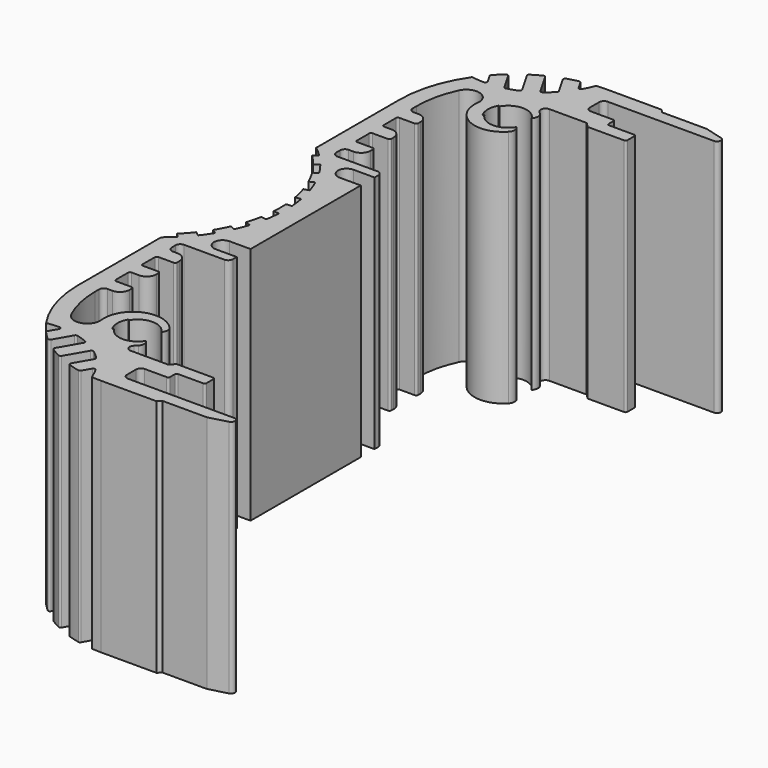
from build123d import *

# Parameters (mm, degrees)
F1_DEPTH = 25


# Not quite as in the source:
# - ends of sketch curves that miss each other by under 0.0002 mm in the source are joined


with BuildPart() as f1:
    # F0 (on Top) → F1 (new body)
    with BuildSketch(Plane.XY):
        with BuildLine():
            ThreePointArc((4.8, 40.2), (3.9, 41.1), (4.8, 42))
            Line((4.8, 42), (7, 42))
            Line((7, 42), (7, 42.5))
            ThreePointArc((7, 42.5), (6.8535533906, 42.8535533906), (6.5, 43))
            Line((6.5, 43), (2.3, 43))
            ThreePointArc((2.3, 43), (1.9464466094, 43.1464466094), (1.8, 43.5))
            Line((1.8, 43.5), (1.8, 44))
            ThreePointArc((1.8, 44), (1.9464466094, 44.3535533906), (2.3, 44.5))
            Line((2.3, 44.5), (2.8, 44.5))
            ThreePointArc((2.8, 44.5), (3.5071067812, 44.7928932188), (3.8, 45.5))
            Line((3.8, 45.5), (3.8, 45.8))
            ThreePointArc((3.8, 45.8), (3.7414213562, 45.9414213562), (3.6, 46))
            Line((3.6, 46), (2, 46))
            ThreePointArc((2, 46), (1.8585786438, 46.0585786438), (1.8, 46.2))
            Line((1.8, 46.2), (1.8, 47.8))
            ThreePointArc((1.8, 47.8), (1.8585786438, 47.9414213562), (2, 48))
            Line((2, 48), (3.6, 48))
            ThreePointArc((3.6, 48), (3.7414213562, 48.0585786438), (3.8, 48.2))
            Line((3.8, 48.2), (3.8, 48.5))
            ThreePointArc((3.8, 48.5), (3.5071067812, 49.2071067812), (2.8, 49.5))
            Line((2.8, 49.5), (2, 49.5))
            ThreePointArc((2, 49.5), (1.8585786438, 49.5585786438), (1.8, 49.7))
            Line((1.8, 49.7), (1.8, 51.3))
            ThreePointArc((1.8, 51.3), (1.8585786438, 51.4414213562), (2, 51.5))
            Line((2, 51.5), (3.6, 51.5))
            ThreePointArc((3.6, 51.5), (3.7414213562, 51.5585786438), (3.8, 51.7))
            Line((3.8, 51.7), (3.8, 52))
            ThreePointArc((3.8, 52), (3.5071067812, 52.7071067812), (2.8, 53))
            Line((2.8, 53), (2.3, 53))
            ThreePointArc((2.3, 53), (1.9464466094, 53.1464466094), (1.8, 53.5))
            Line((1.8, 53.5), (1.8, 54))
            ThreePointArc((1.8, 54), (2.0436001136, 56.2158748388), (2.762764961, 58.3259090183))
            ThreePointArc((2.762764961, 58.3259090183), (4.3620080124, 59.0497497539), (5.3243723966, 57.5816289491))
            ThreePointArc((5.3243723966, 57.5816289491), (7.0286356645, 54.4827159283), (10.4997810009, 55.1601559991))
            ThreePointArc((10.4997810009, 55.1601559991), (10.6996495862, 55.686837824), (10.4765015079, 56.2040865149))
            ThreePointArc((10.4765015079, 56.2040865149), (8.7878814888, 55.2500376563), (7.111250347, 56.2250002003))
            Line((7.111250347, 56.2250002003), (6.981347, 56.15))
            ThreePointArc((6.981347, 56.15), (6.7, 57.2), (6.981346739, 58.2500001507))
            Line((6.981346739, 58.2500001507), (7.11125, 58.175))
            ThreePointArc((7.11125, 58.175), (8.7878814888, 59.1499623437), (10.4765009342, 58.1959139609))
            ThreePointArc((10.4765009342, 58.1959139609), (10.6996495862, 58.713162176), (10.4997811347, 59.2398441249))
            ThreePointArc((10.4997811347, 59.2398441249), (10.3829853135, 59.3589747992), (10.2597477904, 59.471428757))
            ThreePointArc((10.2597477904, 59.471428757), (10.1177123869, 60.0242332623), (10.586373, 60.35))
            Line((10.586373, 60.35), (14.5, 60.35))
            Line((14.5, 60.35), (15, 59.85))
            Line((15, 59.85), (18.8, 59.85))
            ThreePointArc((18.8, 59.85), (18.9414213562, 59.9085786438), (19, 60.05))
            Line((19, 60.05), (19, 60.95))
            ThreePointArc((19, 60.95), (18.9414213562, 61.0914213562), (18.8, 61.15))
            Line((18.8, 61.15), (16.2, 61.15))
            ThreePointArc((16.2, 61.15), (16.0585786438, 61.2085786438), (16, 61.35))
            Line((16, 61.35), (16, 61.95))
            ThreePointArc((16, 61.95), (15.9414213562, 62.0914213562), (15.8, 62.15))
            Line((15.8, 62.15), (13.5, 62.15))
            ThreePointArc((13.5, 62.15), (13.1464466094, 62.2964466094), (13, 62.65))
            Line((13, 62.65), (13, 63.85))
            ThreePointArc((13, 63.85), (13.1464466094, 64.2035533906), (13.5, 64.35))
            Line((13.5, 64.35), (24.6, 64.35))
            ThreePointArc((24.6, 64.35), (24.9965779149, 64.6977892978), (24.703528057, 65.1363702129))
            Line((24.703528057, 65.1363702129), (22.786636, 65.65))
            Line((22.786636, 65.65), (18.15, 65.65))
            Line((18.15, 65.65), (17.8, 66))
            Line((17.8, 66), (12, 66))
            ThreePointArc((12, 66), (11.5037956196, 65.9897364947), (11.0084400385, 65.9589635355))
            ThreePointArc((11.0084400385, 65.9589635355), (10.7579980706, 65.3552616733), (10.4591110079, 64.7740179955))
            ThreePointArc((10.4591110079, 64.7740179955), (10.2859108214, 64.6726695125), (10.1119279394, 64.772667965))
            Line((10.1119279394, 64.772667965), (9.622174, 65.620948))
            ThreePointArc((9.622174, 65.620948), (9.5295416944, 65.704000017), (9.4057309446, 65.7162182501))
            ThreePointArc((9.4057309446, 65.7162182501), (8.8440365093, 65.5775599521), (8.2896780658, 65.4119897978))
            ThreePointArc((8.2896780658, 65.4119897978), (8.1647942155, 65.2934461354), (8.1783119394, 65.121789965))
            Line((8.1783119394, 65.121789965), (9.213226, 63.329266))
            ThreePointArc((9.213226, 63.329266), (9.2383677655, 63.2036035638), (9.1820724438, 63.0884775512))
            ThreePointArc((9.1820724438, 63.0884775512), (8.7626678335, 62.6946927651), (8.316047761, 62.3320673169))
            ThreePointArc((8.316047761, 62.3320673169), (8.1557959784, 62.2957762661), (8.0224409394, 62.391765965))
            Line((8.0224409394, 62.391765965), (6.757013, 64.583552))
            ThreePointArc((6.757013, 64.583552), (6.6400709156, 64.6754751209), (6.4920078967, 64.6612392))
            ThreePointArc((6.4920078967, 64.6612392), (6.0000000485, 64.3923048734), (5.5210921245, 64.1006808058))
            ThreePointArc((5.5210921245, 64.1006808058), (5.4347322038, 63.9795722811), (5.4558689394, 63.832335965))
            Line((5.4558689394, 63.832335965), (6.721447, 61.640291))
            ThreePointArc((6.721447, 61.640291), (6.737909119, 61.4768372061), (6.6264020443, 61.3561958956))
            ThreePointArc((6.6264020443, 61.3561958956), (6.0891473301, 61.1505669893), (5.5385048838, 60.984077441))
            ThreePointArc((5.5385048838, 60.984077441), (5.4106226111, 60.9928590787), (5.3143369394, 61.077475965))
            Line((5.3143369394, 61.077475965), (4.279091, 62.870574))
            ThreePointArc((4.279091, 62.870574), (4.1371914661, 62.9681087255), (3.9720878604, 62.9192281551))
            ThreePointArc((3.9720878604, 62.9192281551), (3.5515207716, 62.5219245906), (3.1505919848, 62.1048120139))
            ThreePointArc((3.1505919848, 62.1048120139), (3.0992679352, 61.9914798188), (3.1248769394, 61.869731965))
            Line((3.1248769394, 61.869731965), (3.615346, 61.020215))
            ThreePointArc((3.615346, 61.020215), (3.6149741489, 60.8195735441), (3.4406580037, 60.7202204983))
            ThreePointArc((3.4406580037, 60.7202204983), (2.7869604683, 60.7518399473), (2.138034956, 60.8367867453))
            ThreePointArc((2.138034956, 60.8367867453), (0.5469747265, 57.5816493525), (0, 54))
            Line((0, 54), (0, 43.132527))
            ThreePointArc((0, 43.132527), (0.5182749816, 42.7008809568), (1.013299072, 42.2427560738))
            Line((1.013299072, 42.2427560738), (0.608364, 41.827512))
            ThreePointArc((0.608364, 41.827512), (1.1629757499, 41.2503803189), (1.6789731577, 40.6384801245))
            Line((1.6789731577, 40.6384801245), (2.134269, 40.997792))
            ThreePointArc((2.134269, 40.997792), (2.5752529618, 40.4048716933), (2.9815908821, 39.7876919271))
            Line((2.9815908821, 39.7876919271), (2.488227, 39.482745))
            ThreePointArc((2.488227, 39.482745), (2.886743943, 38.7885841377), (3.2393819334, 38.0700289699))
            Line((3.2393819334, 38.0700289699), (3.768079, 38.308522))
            ThreePointArc((3.768079, 38.308522), (4.0525233611, 37.6265300852), (4.2974820523, 36.9293810167))
            Line((4.2974820523, 36.9293810167), (3.745, 36.752848))
            ThreePointArc((3.745, 36.752848), (3.9637463545, 35.982896774), (4.1320752415, 35.2003750438))
            Line((4.1320752415, 35.2003750438), (4.702765, 35.30388))
            ThreePointArc((4.702765, 35.30388), (4.8137708235, 34.5733331759), (4.8827975487, 33.8376319707))
            Line((4.8827975487, 33.8376319707), (4.30402, 33.8))
            ThreePointArc((4.30402, 33.8), (4.33, 33), (4.3040196698, 32.2000000215))
            Line((4.3040196698, 32.2000000215), (4.882798, 32.162368))
            ThreePointArc((4.882798, 32.162368), (4.8137708235, 31.4266668241), (4.7027649352, 30.6961200117))
            Line((4.7027649352, 30.6961200117), (4.132075, 30.799625))
            ThreePointArc((4.132075, 30.799625), (3.9637463545, 30.017103226), (3.7450002661, 29.247151915))
            Line((3.7450002661, 29.247151915), (4.297482, 29.070619))
            ThreePointArc((4.297482, 29.070619), (4.0525233611, 28.3734699148), (3.7680793822, 27.6914778276))
            Line((3.7680793822, 27.6914778276), (3.239382, 27.929971))
            ThreePointArc((3.239382, 27.929971), (2.886743943, 27.2114158623), (2.4882274023, 26.5172547514))
            Line((2.4882274023, 26.5172547514), (2.981591, 26.212308))
            ThreePointArc((2.981591, 26.212308), (2.5752529618, 25.5951283067), (2.1342694548, 25.0022076411))
            Line((2.1342694548, 25.0022076411), (1.678973, 25.36152))
            ThreePointArc((1.678973, 25.36152), (1.1629757499, 24.7496196811), (0.6083640321, 24.1724879671))
            Line((0.6083640321, 24.1724879671), (1.013299, 23.757244))
            ThreePointArc((1.013299, 23.757244), (0.5182749816, 23.2991190432), (-8.17e-08, 22.8674731035))
            Line((-8.17e-08, 22.8674731035), (0, 12))
            ThreePointArc((0, 12), (0.5469747265, 8.4183506475), (2.1380353474, 5.1632132408))
            ThreePointArc((2.1380353474, 5.1632132408), (2.7869604683, 5.2481600527), (3.4406580007, 5.2797799049))
            ThreePointArc((3.4406580007, 5.2797799049), (3.6149741489, 5.1804264559), (3.6153460606, 4.979784965))
            Line((3.6153460606, 4.979784965), (3.124877, 4.130268))
            ThreePointArc((3.124877, 4.130268), (3.0992679352, 4.0085201812), (3.1505918276, 3.8951878421))
            ThreePointArc((3.1505918276, 3.8951878421), (3.5515207716, 3.4780754094), (3.9720879776, 3.0807719751))
            ThreePointArc((3.9720879776, 3.0807719751), (4.1371914661, 3.0318912745), (4.2790910606, 3.129425965))
            Line((4.2790910606, 3.129425965), (5.314337, 4.922524))
            ThreePointArc((5.314337, 4.922524), (5.4106226111, 5.0071409213), (5.5385047448, 5.0159220316))
            ThreePointArc((5.5385047448, 5.0159220316), (6.0891473301, 4.8494330107), (6.6264020289, 4.6438040681))
            ThreePointArc((6.6264020289, 4.6438040681), (6.737909119, 4.5231627939), (6.7214470606, 4.359708965))
            Line((6.7214470606, 4.359708965), (5.455869, 2.167664))
            ThreePointArc((5.455869, 2.167664), (5.4347322038, 2.0204277189), (5.5210922043, 1.8993193185))
            ThreePointArc((5.5210922043, 1.8993193185), (6.0000000485, 1.6076951266), (6.492007864, 1.3387607367))
            ThreePointArc((6.492007864, 1.3387607367), (6.6400709156, 1.3245248791), (6.7570130606, 1.416447965))
            Line((6.7570130606, 1.416447965), (8.022441, 3.608234))
            ThreePointArc((8.022441, 3.608234), (8.1557959784, 3.7042237339), (8.3160473796, 3.6679321771))
            ThreePointArc((8.3160473796, 3.6679321771), (8.7626678335, 3.3053072349), (9.1820727835, 2.9115227854))
            ThreePointArc((9.1820727835, 2.9115227854), (9.2383677655, 2.7963964362), (9.2132260606, 2.670733965))
            Line((9.2132260606, 2.670733965), (8.178312, 0.87821))
            ThreePointArc((8.178312, 0.87821), (8.1647942155, 0.7065538646), (8.2896780788, 0.5880102423))
            ThreePointArc((8.2896780788, 0.5880102423), (8.8440365093, 0.4224400479), (9.4057309628, 0.2837818319))
            ThreePointArc((9.4057309628, 0.2837818319), (9.5295416944, 0.295999983), (9.6221740606, 0.379051965))
            Line((9.6221740606, 0.379051965), (10.111928, 1.227332))
            ThreePointArc((10.111928, 1.227332), (10.2859108214, 1.3273304875), (10.4591106369, 1.2259817941))
            ThreePointArc((10.4591106369, 1.2259817941), (10.7579980706, 0.6447383267), (11.0084405264, 0.0410361936))
            ThreePointArc((11.0084405264, 0.0410361936), (11.5037956196, 0.0102635053), (12, 0))
            Line((12, 0), (17.8, 0))
            Line((17.8, 0), (18.15, 0.35))
            Line((18.15, 0.35), (22.786636, 0.35))
            Line((22.786636, 0.35), (24.703528, 0.86363))
            ThreePointArc((24.703528, 0.86363), (24.9965779149, 1.3022107022), (24.6, 1.65))
            Line((24.6, 1.65), (13.5, 1.65))
            ThreePointArc((13.5, 1.65), (13.1464466094, 1.7964466094), (13, 2.15))
            Line((13, 2.15), (13, 3.35))
            ThreePointArc((13, 3.35), (13.1464466094, 3.7035533906), (13.5, 3.85))
            Line((13.5, 3.85), (15.8, 3.85))
            ThreePointArc((15.8, 3.85), (15.9414213562, 3.9085786438), (16, 4.05))
            Line((16, 4.05), (16, 4.65))
            ThreePointArc((16, 4.65), (16.0585786438, 4.7914213562), (16.2, 4.85))
            Line((16.2, 4.85), (18.8, 4.85))
            ThreePointArc((18.8, 4.85), (18.9414213562, 4.9085786438), (19, 5.05))
            Line((19, 5.05), (19, 5.95))
            ThreePointArc((19, 5.95), (18.9414213562, 6.0914213562), (18.8, 6.15))
            Line((18.8, 6.15), (15, 6.15))
            Line((15, 6.15), (14.5, 5.65))
            Line((14.5, 5.65), (10.586373, 5.65))
            ThreePointArc((10.586373, 5.65), (10.1177123869, 5.9757667377), (10.2597479299, 6.5285710813))
            ThreePointArc((10.2597479299, 6.5285710813), (10.3829853135, 6.6410252008), (10.4997810009, 6.7601559991))
            ThreePointArc((10.4997810009, 6.7601559991), (10.6996495862, 7.286837824), (10.4765015079, 7.8040865149))
            ThreePointArc((10.4765015079, 7.8040865149), (8.7878814888, 6.8500376563), (7.111250347, 7.8250002003))
            Line((7.111250347, 7.8250002003), (6.981347, 7.75))
            ThreePointArc((6.981347, 7.75), (6.7, 8.8), (6.981346739, 9.8500001507))
            Line((6.981346739, 9.8500001507), (7.11125, 9.775))
            ThreePointArc((7.11125, 9.775), (8.7878814888, 10.7499623437), (10.4765009342, 9.7959139609))
            ThreePointArc((10.4765009342, 9.7959139609), (10.6996495862, 10.313162176), (10.4997811347, 10.8398441249))
            ThreePointArc((10.4997811347, 10.8398441249), (7.0286356645, 11.5172840717), (5.3243724444, 8.418371057))
            ThreePointArc((5.3243724444, 8.418371057), (4.3620080124, 6.9502502461), (2.7627648987, 7.6740909525))
            ThreePointArc((2.7627648987, 7.6740909525), (2.0436001136, 9.7841251612), (1.8, 12))
            Line((1.8, 12), (1.8, 12.5))
            ThreePointArc((1.8, 12.5), (1.9464466094, 12.8535533906), (2.3, 13))
            Line((2.3, 13), (2.8, 13))
            ThreePointArc((2.8, 13), (3.5071067812, 13.2928932188), (3.8, 14))
            Line((3.8, 14), (3.8, 14.3))
            ThreePointArc((3.8, 14.3), (3.7414213562, 14.4414213562), (3.6, 14.5))
            Line((3.6, 14.5), (2, 14.5))
            ThreePointArc((2, 14.5), (1.8585786438, 14.5585786438), (1.8, 14.7))
            Line((1.8, 14.7), (1.8, 16.3))
            ThreePointArc((1.8, 16.3), (1.8585786438, 16.4414213562), (2, 16.5))
            Line((2, 16.5), (2.8, 16.5))
            ThreePointArc((2.8, 16.5), (3.5071067812, 16.7928932188), (3.8, 17.5))
            Line((3.8, 17.5), (3.8, 17.8))
            ThreePointArc((3.8, 17.8), (3.7414213562, 17.9414213562), (3.6, 18))
            Line((3.6, 18), (2, 18))
            ThreePointArc((2, 18), (1.8585786438, 18.0585786438), (1.8, 18.2))
            Line((1.8, 18.2), (1.8, 19.8))
            ThreePointArc((1.8, 19.8), (1.8585786438, 19.9414213562), (2, 20))
            Line((2, 20), (3.6, 20))
            ThreePointArc((3.6, 20), (3.7414213562, 20.0585786438), (3.8, 20.2))
            Line((3.8, 20.2), (3.8, 20.5))
            ThreePointArc((3.8, 20.5), (3.5071067812, 21.2071067812), (2.8, 21.5))
            Line((2.8, 21.5), (2.3, 21.5))
            ThreePointArc((2.3, 21.5), (1.9464466094, 21.6464466094), (1.8, 22))
            Line((1.8, 22), (1.8, 22.5))
            ThreePointArc((1.8, 22.5), (1.9464466094, 22.8535533906), (2.3, 23))
            Line((2.3, 23), (6.5, 23))
            ThreePointArc((6.5, 23), (6.8535533906, 23.1464466094), (7, 23.5))
            Line((7, 23.5), (7, 24))
            Line((7, 24), (4.8, 24))
            ThreePointArc((4.8, 24), (3.9, 24.9), (4.8, 25.8))
            Line((4.8, 25.8), (7, 25.8))
            Line((7, 25.8), (7, 40.2))
            Line((7, 40.2), (4.8, 40.2))
        make_face()
    extrude(amount=F1_DEPTH)


solid = f1.part
